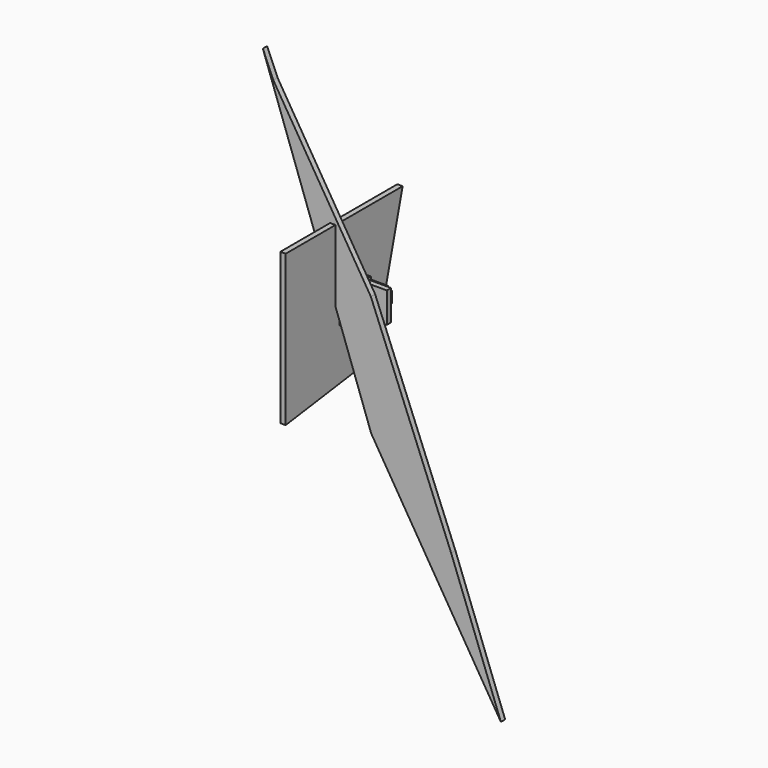
from build123d import *

# Parameters (mm, degrees)
F1_DEPTH = 25.4
F3_DEPTH = 25.4
F4_W     = 29.7458320856
F4_H     = 10.7239410281
F4_W_2   = 77.620446682
F4_W_3   = 25.7802940905
F4_H_2   = 64.6573156118
F4_W_4   = 82.3989063501
F4_H_3   = 15.7408937812
F4_W_5   = 43.0548340082
F4_H_4   = 22.1842341125
F4_W_6   = 2.0285844803
F4_H_5   = 2.3600235581
F5_DEPTH = 25.4
F7_DEPTH = 25.4


with BuildPart() as f1:
    # F0 (on Front) → F1 (new body)
    with BuildSketch(Plane.XZ):
        Polygon((90.7035768032, 111.3269925117), (-373.5082440503, 867.1883240136), (-423.3669042587, 983.7029576302), (92.4958586693, -462.0907306671), (710.130751133, -1470.7733392715), (473.2221364975, -839.5437598228), align=None)
    extrude(amount=F1_DEPTH)

    # F2 (on face) → F3 (join)
    with BuildSketch(Plane(origin=(0, 0, 0), x_dir=(-1, 0, 0), z_dir=(0, 1, 0))):
        Polygon((-81.9063782692, 78.366830945), (-73.3345150948, 78.366830945), (-73.3345150948, 75.38125664), (0, 75.38125664), (0, 144.7913646698), (-146.6690301895, 144.7913646698), (-146.6690301895, 0), (-77.620446682, 0), (-77.620446682, 72.3956823349), (-81.9063782692, 72.3956823349), align=None)
        Polygon((0, 75.38125664), (-73.3345150948, 75.38125664), (-73.3345150948, 72.3956823349), (-77.620446682, 72.3956823349), (-77.620446682, 0), (0, 0), align=None)
        Polygon((77.620446682, 75.38125664), (0, 75.38125664), (0, 0), (-77.620446682, 0), (-77.620446682, -75.38125664), (77.620446682, -75.38125664), align=None)
    extrude(amount=F3_DEPTH)

    # F4 (on face) → F5 (join)
    with BuildSketch(Plane(origin=(0, 25.4, 0), x_dir=(-1, 0, 0), z_dir=(0, 1, 0))):
        with Locations((-14.8729160428, 70.0192861259)):
            Rectangle(F4_W, F4_H)
        Polygon((-43.309610337, 64.6573156118), (-29.7458320856, 64.6573156118), (-29.7458320856, 75.38125664), (-29.7458320856, 116.2622794509), (-112.1447384357, 116.2622794509), (-112.1447384357, 64.6573156118), (-69.0899044275, 64.6573156118), align=None)
        Polygon((0, 64.6573156118), (-29.7458320856, 64.6573156118), (-43.309610337, 64.6573156118), (-43.309610337, 0), (-43.309610337, -75.38125664), (77.620446682, -75.38125664), (77.620446682, 64.6573156118), align=None)
        with Locations((38.810223341, 70.0192861259)):
            Rectangle(F4_W_2, F4_H)
        Polygon((-29.7458320856, 116.2622794509), (-29.7458320856, 75.38125664), (0, 75.38125664), (0, 144.7913646698), (-29.7458320856, 144.7913646698), (-29.7458320856, 132.0031732321), align=None)
        with Locations((-56.1997573823, 32.3286578059)):
            Rectangle(F4_W_3, F4_H_2)
        with Locations((-70.9452852607, 124.1327263415)):
            Rectangle(F4_W_4, F4_H_3)
        with Locations((-90.6173214316, 32.3286578059)):
            Rectangle(F4_W_5, F4_H_2)
        Polygon((-112.1447384357, 64.6573156118), (-112.1447384357, 116.2622794509), (-128.1245350838, 116.2622794509), (-130.1531195641, 116.2622794509), (-130.1531195641, 64.6573156118), align=None)
        with Locations((-90.6173214316, -11.0921170563)):
            Rectangle(F4_W_5, F4_H_4)
        with Locations((-129.1388273239, 117.44229123)):
            Rectangle(F4_W_6, F4_H_5)
    extrude(amount=F5_DEPTH)

    # F6 (on face) → F7 (join)
    with BuildSketch(Plane(origin=(-77.620446682, 0, 0), x_dir=(0, -1, 0), z_dir=(-1, 0, 0))):
        Polygon((321.7040300369, 356.4623594284), (-374.66776371, 356.4623594284), (-204.5531272888, -290.0140881538), (321.7040300369, -362.3423576355), align=None)
    extrude(amount=F7_DEPTH)


solid = f1.part
